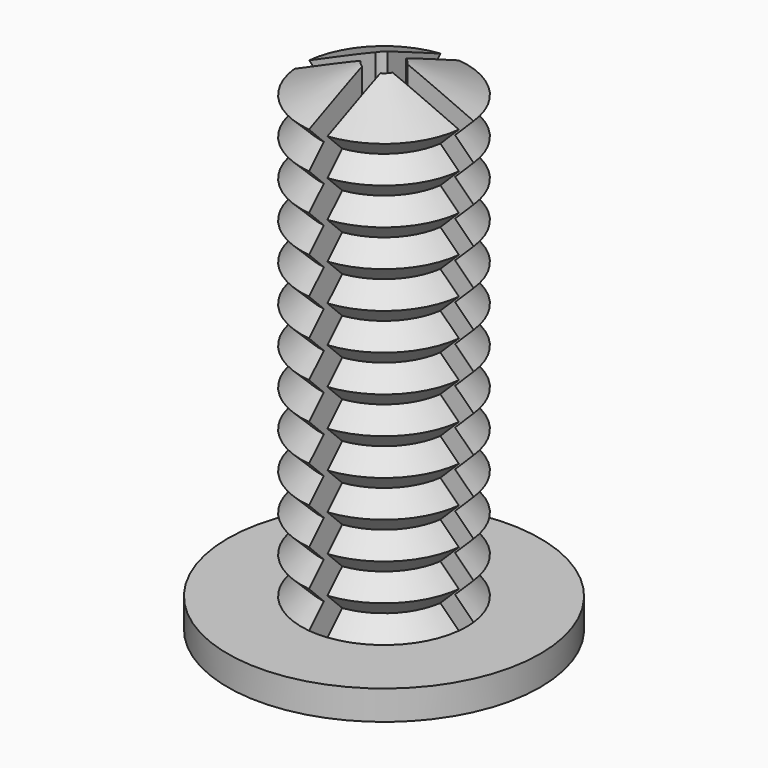
from build123d import *

# Parameters (mm, degrees)
F1_R     = 4.25
F4_DEPTH = 0.8
F5_DEPTH = 13.001
F6_DEPTH = 25


with BuildPart() as f3:
    # F2 (on Front) → F3 (revolve)
    with BuildSketch(Plane.XZ):
        Polygon((-1.75, 0.5), (-2.25, 0), (0, 0), (0, 13), (-2.25, 12), (-1.75, 11.5), (-2.25, 11), (-1.75, 10.5), (-2.25, 10), (-1.75, 9.5), (-2.25, 9), (-1.75, 8.5), (-2.25, 8), (-1.75, 7.5), (-2.25, 7), (-1.75, 6.5), (-2.25, 6), (-1.75, 5.5), (-2.25, 5), (-1.75, 4.5), (-2.25, 4), (-1.75, 3.5), (-2.25, 3), (-1.75, 2.5), (-2.25, 2), (-1.75, 1.5), (-2.25, 1), align=None)
    revolve(axis=Axis((0, 0, 6.5), (0, 0, 1)))

    # F1 (on Top) → F4 (join)
    with BuildSketch(Plane.XY):
        Circle(F1_R)
        with BuildLine():
            ThreePointArc((2.2360679775, 0.25), (2.2465142943, 0.1251939508), (2.25, 0))
            ThreePointArc((2.25, 0), (2.2465142943, -0.1251939508), (2.2360679775, -0.25))
            ThreePointArc((2.2360679775, -0.25), (1.5909902577, -1.5909902577), (0.25, -2.2360679775))
            ThreePointArc((0.25, -2.2360679775), (0, -2.25), (-0.25, -2.2360679775))
            ThreePointArc((-0.25, -2.2360679775), (-1.5909902577, -1.5909902577), (-2.2360679775, -0.25))
            ThreePointArc((-2.2360679775, -0.25), (-2.25, 0), (-2.2360679775, 0.25))
            ThreePointArc((-2.2360679775, 0.25), (-1.5909902577, 1.5909902577), (-0.25, 2.2360679775))
            ThreePointArc((-0.25, 2.2360679775), (0, 2.25), (0.25, 2.2360679775))
            ThreePointArc((0.25, 2.2360679775), (1.5909902577, 1.5909902577), (2.2360679775, 0.25))
        make_face(mode=Mode.SUBTRACT)
        with BuildLine():
            Line((0.4330127019, 0.25), (2.2360679775, 0.25))
            ThreePointArc((2.2360679775, 0.25), (1.5909902577, 1.5909902577), (0.25, 2.2360679775))
            Line((0.25, 2.2360679775), (0.25, 0.4330127019))
            ThreePointArc((0.25, 0.4330127019), (0.3535533906, 0.3535533906), (0.4330127019, 0.25))
        make_face()
        with BuildLine():
            ThreePointArc((0.25, -2.2360679775), (1.5909902577, -1.5909902577), (2.2360679775, -0.25))
            Line((2.2360679775, -0.25), (0.4330127019, -0.25))
            ThreePointArc((0.4330127019, -0.25), (0.3535533906, -0.3535533906), (0.25, -0.4330127019))
            Line((0.25, -0.4330127019), (0.25, -2.2360679775))
        make_face()
        with BuildLine():
            Line((-0.25, 0.4330127019), (-0.25, 2.2360679775))
            ThreePointArc((-0.25, 2.2360679775), (-1.5909902577, 1.5909902577), (-2.2360679775, 0.25))
            Line((-2.2360679775, 0.25), (-0.4330127019, 0.25))
            ThreePointArc((-0.4330127019, 0.25), (-0.3535533906, 0.3535533906), (-0.25, 0.4330127019))
        make_face()
        with BuildLine():
            ThreePointArc((-2.2360679775, -0.25), (-1.5909902577, -1.5909902577), (-0.25, -2.2360679775))
            Line((-0.25, -2.2360679775), (-0.25, -0.4330127019))
            ThreePointArc((-0.25, -0.4330127019), (-0.3535533906, -0.3535533906), (-0.4330127019, -0.25))
            Line((-0.4330127019, -0.25), (-2.2360679775, -0.25))
        make_face()
    extrude(amount=-F4_DEPTH)

    # F1 (on Top) → F5 (cut, through all)
    with BuildSketch(Plane.XY):
        with BuildLine():
            ThreePointArc((0.5, 0), (0.4829629131, 0.1294095226), (0.4330127019, 0.25))
            ThreePointArc((0.4330127019, 0.25), (0.3535533906, 0.3535533906), (0.25, 0.4330127019))
            ThreePointArc((0.25, 0.4330127019), (0, 0.5), (-0.25, 0.4330127019))
            ThreePointArc((-0.25, 0.4330127019), (-0.3535533906, 0.3535533906), (-0.4330127019, 0.25))
            ThreePointArc((-0.4330127019, 0.25), (-0.5, 0), (-0.4330127019, -0.25))
            ThreePointArc((-0.4330127019, -0.25), (-0.3535533906, -0.3535533906), (-0.25, -0.4330127019))
            ThreePointArc((-0.25, -0.4330127019), (0, -0.5), (0.25, -0.4330127019))
            ThreePointArc((0.25, -0.4330127019), (0.3535533906, -0.3535533906), (0.4330127019, -0.25))
            ThreePointArc((0.4330127019, -0.25), (0.4829629131, -0.1294095226), (0.5, 0))
        make_face()
        with BuildLine():
            Line((-0.4330127019, 0.25), (-2.2360679775, 0.25))
            ThreePointArc((-2.2360679775, 0.25), (-2.25, 0), (-2.2360679775, -0.25))
            Line((-2.2360679775, -0.25), (-0.4330127019, -0.25))
            ThreePointArc((-0.4330127019, -0.25), (-0.5, 0), (-0.4330127019, 0.25))
        make_face()
        with BuildLine():
            Line((0.25, 0.4330127019), (0.25, 2.2360679775))
            ThreePointArc((0.25, 2.2360679775), (0, 2.25), (-0.25, 2.2360679775))
            Line((-0.25, 2.2360679775), (-0.25, 0.4330127019))
            ThreePointArc((-0.25, 0.4330127019), (0, 0.5), (0.25, 0.4330127019))
        make_face()
        with BuildLine():
            ThreePointArc((2.2360679775, -0.25), (2.2465142943, -0.1251939508), (2.25, 0))
            ThreePointArc((2.25, 0), (2.2465142943, 0.1251939508), (2.2360679775, 0.25))
            Line((2.2360679775, 0.25), (0.4330127019, 0.25))
            ThreePointArc((0.4330127019, 0.25), (0.4829629131, 0.1294095226), (0.5, 0))
            ThreePointArc((0.5, 0), (0.4829629131, -0.1294095226), (0.4330127019, -0.25))
            Line((0.4330127019, -0.25), (2.2360679775, -0.25))
        make_face()
        with BuildLine():
            ThreePointArc((-0.25, -2.2360679775), (0, -2.25), (0.25, -2.2360679775))
            Line((0.25, -2.2360679775), (0.25, -0.4330127019))
            ThreePointArc((0.25, -0.4330127019), (0, -0.5), (-0.25, -0.4330127019))
            Line((-0.25, -0.4330127019), (-0.25, -2.2360679775))
        make_face()
    extrude(amount=F5_DEPTH, mode=Mode.SUBTRACT)

    # F1 (on Top) → F6 (cut)
    with BuildSketch(Plane.XY):
        with BuildLine():
            Line((-0.4330127019, 0.25), (-2.2360679775, 0.25))
            ThreePointArc((-2.2360679775, 0.25), (-2.25, 0), (-2.2360679775, -0.25))
            Line((-2.2360679775, -0.25), (-0.4330127019, -0.25))
            ThreePointArc((-0.4330127019, -0.25), (-0.5, 0), (-0.4330127019, 0.25))
        make_face()
        with BuildLine():
            ThreePointArc((-0.25, -2.2360679775), (0, -2.25), (0.25, -2.2360679775))
            Line((0.25, -2.2360679775), (0.25, -0.4330127019))
            ThreePointArc((0.25, -0.4330127019), (0, -0.5), (-0.25, -0.4330127019))
            Line((-0.25, -0.4330127019), (-0.25, -2.2360679775))
        make_face()
        with BuildLine():
            ThreePointArc((2.2360679775, -0.25), (2.2465142943, -0.1251939508), (2.25, 0))
            ThreePointArc((2.25, 0), (2.2465142943, 0.1251939508), (2.2360679775, 0.25))
            Line((2.2360679775, 0.25), (0.4330127019, 0.25))
            ThreePointArc((0.4330127019, 0.25), (0.4829629131, 0.1294095226), (0.5, 0))
            ThreePointArc((0.5, 0), (0.4829629131, -0.1294095226), (0.4330127019, -0.25))
            Line((0.4330127019, -0.25), (2.2360679775, -0.25))
        make_face()
        with BuildLine():
            Line((0.25, 0.4330127019), (0.25, 2.2360679775))
            ThreePointArc((0.25, 2.2360679775), (0, 2.25), (-0.25, 2.2360679775))
            Line((-0.25, 2.2360679775), (-0.25, 0.4330127019))
            ThreePointArc((-0.25, 0.4330127019), (0, 0.5), (0.25, 0.4330127019))
        make_face()
    extrude(amount=-F6_DEPTH, mode=Mode.SUBTRACT)


solid = f3.part
